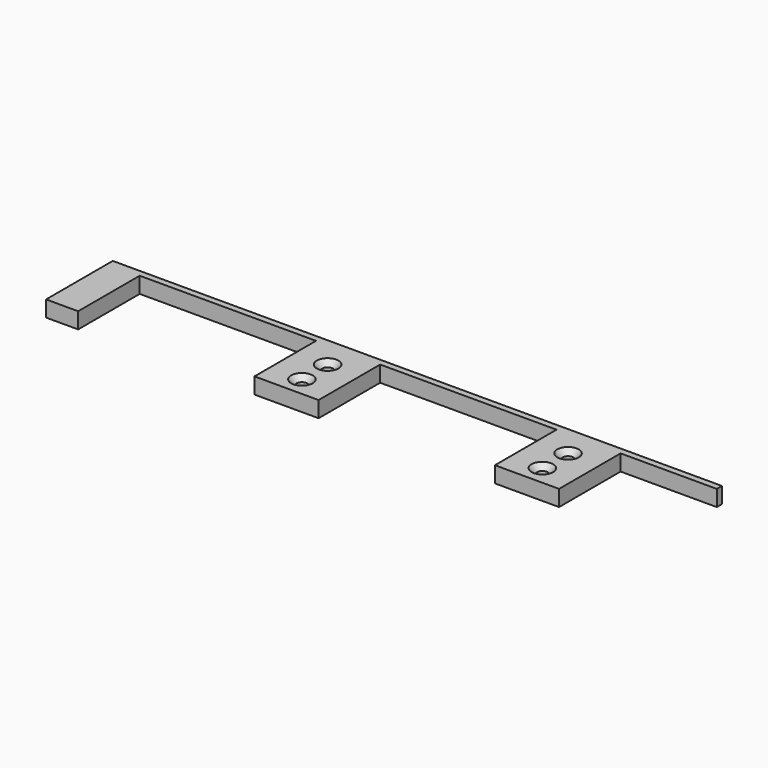
from build123d import *

# Parameters (mm, degrees)
F0_R           = 1.7
F1_DEPTH       = 5
F3_D           = 3.4
F3_CSINK_D     = 6.72
F3_CSINK_ANGLE = 90


with BuildPart() as f1:
    # F0 (on Top) → F1 (new body)
    with BuildSketch(Plane.XY):
        Polygon((95, 13), (-95, 13), (-95, -13), (-85, -13), (-85, 11), (-30, 11), (-30, 3), (-30, -13), (-10, -13), (-10, 11), (45, 11), (45, 3), (45, -13), (65, -13), (65, 11), (95, 11), align=None)
        with Locations((-20, -7)):
            Circle(F0_R, mode=Mode.SUBTRACT)
        with Locations((55, -7)):
            Circle(F0_R, mode=Mode.SUBTRACT)
        with Locations((-20, 3)):
            Circle(F0_R, mode=Mode.SUBTRACT)
        with Locations((55, 3)):
            Circle(F0_R, mode=Mode.SUBTRACT)
    extrude(amount=F1_DEPTH)

    # F3 (through all)
    with Locations(Plane.XY.offset(5)):
        with Locations((-20, 3), (-20, -7), (55, 3), (55, -7)):
            CounterSinkHole(F3_D / 2, F3_CSINK_D / 2, counter_sink_angle=F3_CSINK_ANGLE)


solid = f1.part
